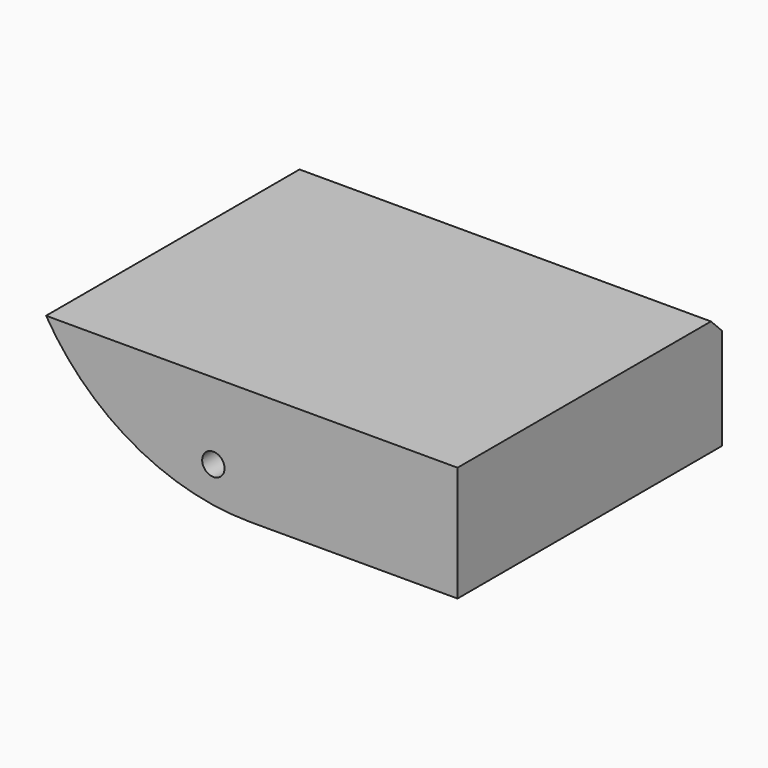
from build123d import *

# Parameters (mm, degrees)
F0_W        = 150
F0_H        = 120.4859416558
F1_DEPTH    = 42
F2_SIZE     = 5
F3_T1_DEPTH = 492.526994922
F6_R        = 4.0747978112
F7_DEPTH    = 192


# Not quite as in the source:
# - a fillet or chamfer that OpenCascade refuses, or shapes differently, is made with other operations: its cross-section is extruded or revolved along the edge and cut away or added
# - the program builds the solid bodies; features that only make, move or delete a surface that nothing else refers to are left out


with BuildPart() as f1:
    # F0 (on Top) → F1 (new body)
    with BuildSketch(Plane.XY):
        with Locations((-21.8634653855, -60.2429708279)):
            Rectangle(F0_W, F0_H)
    extrude(amount=F1_DEPTH)

    # F2
    f2_edges = [f1.edges().sort_by_distance(p)[0] for p in [
        (-21.863465, 0, 42),
    ]]
    chamfer(f2_edges, length=F2_SIZE)

    # F3: fillet of radius 86.9116882454 on 1 edges, made by hand

    # F3_s2 → F3_t1 (cut)
    with BuildSketch(Plane.XZ.offset(-186.0205266331)):
        with BuildLine():
            ThreePointArc((-22.4552547323, 0), (-65.1769758253, 11.2248591368), (-96.8634653855, 42))
            Line((-96.8634653855, 42), (-96.8634653855, 0))
            Line((-96.8634653855, 0), (-22.4552547323, 0))
        make_face()
    extrude(amount=F3_T1_DEPTH, mode=Mode.SUBTRACT)

    # F6 (on face) → F7 (cut)
    with BuildSketch(Plane.XZ.offset(120.4859416558)):
        with Locations((-35.8820706606, 14.1489794478)):
            Circle(F6_R)
    extrude(amount=-F7_DEPTH, mode=Mode.SUBTRACT)


solid = f1.part
